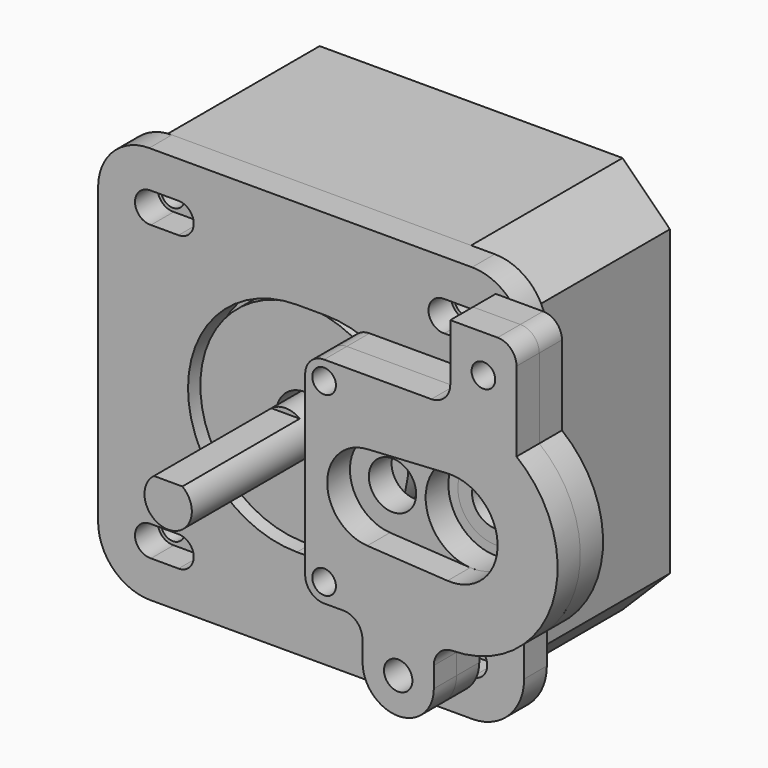
from build123d import *

# Parameters (mm, degrees)
F0_W      = 42
F0_H      = 42
F0_R      = 1.25
F0_R_2    = 11
F0_R_3    = 3
F1_DEPTH  = 20
F2_DEPTH  = 2
F3_SIZE   = 5
F4_R      = 2.5
F5_DEPTH  = 40
F7_DEPTH  = 15.5
F9_DEPTH  = 3
F10_R     = 4
F11_DEPTH = 25
F12_R     = 4
F12_R_2   = 2.5
F13_DEPTH = 2.5
F14_R     = 1.5
F14_R_2   = 2.5
F14_R_3   = 5
F15_DEPTH = 3
F16_R     = 1.5
F17_DEPTH = 3
F18_R     = 1.25
F19_DEPTH = 25


with BuildPart() as f1:
    # F0 (on Front) → F1 (new body)
    with BuildSketch(Plane.XZ):
        Rectangle(F0_W, F0_H)
        with Locations((-15.5, -15.5)):
            Circle(F0_R, mode=Mode.SUBTRACT)
        with Locations((15.5, -15.5)):
            Circle(F0_R, mode=Mode.SUBTRACT)
        with Locations((-15.5, 15.5)):
            Circle(F0_R, mode=Mode.SUBTRACT)
        Circle(F0_R_2, mode=Mode.SUBTRACT)
        with Locations((15.5, 15.5)):
            Circle(F0_R, mode=Mode.SUBTRACT)
        Circle(F0_R_2)
        Circle(F0_R_3, mode=Mode.SUBTRACT)
    extrude(amount=-F1_DEPTH)

    # F0 (on Front) → F2 (join)
    with BuildSketch(Plane.XZ):
        Circle(F0_R_2)
        Circle(F0_R_3, mode=Mode.SUBTRACT)
    extrude(amount=F2_DEPTH)

    # F3
    f3_edges = [f1.edges().sort_by_distance(p)[0] for p in [
        (-21, 10, 21),
        (21, 10, 21),
        (21, 10, -21),
        (-21, 10, -21),
    ]]
    chamfer(f3_edges, length=F3_SIZE)


with BuildPart() as f5:
    # F4 (on face) → F5 (new body)
    with BuildSketch(Plane(origin=(0, 20, 0), x_dir=(-1, 0, 0), z_dir=(0, 1, 0))):
        Circle(F4_R)
    extrude(amount=-F5_DEPTH)

    # F6 (on face) → F7 (cut)
    with BuildSketch(Plane.XZ.offset(20)):
        with BuildLine():
            ThreePointArc((1.5, 2), (0, 2.5), (-1.5, 2))
            Line((-1.5, 2), (1.5, 2))
        make_face()
    extrude(amount=-F7_DEPTH, mode=Mode.SUBTRACT)


with BuildPart() as f9:
    # F8 (on face) → F9 (new body)
    with BuildSketch(Plane.XZ):
        with BuildLine():
            Line((-15.5, -21), (18.5, -21))
            ThreePointArc((18.5, -21), (22.3890872965, -19.3890872965), (24, -15.5))
            Line((24, -15.5), (24, -6.8738635424))
            ThreePointArc((24, -6.8738635424), (28.5, 0), (24, 6.8738635424))
            Line((24, 6.8738635424), (24, 15.5))
            ThreePointArc((24, 15.5), (22.3890872965, 19.3890872965), (18.5, 21))
            Line((18.5, 21), (-15.6, 21))
            ThreePointArc((-15.6, 21), (-19.4183766184, 19.4183766184), (-21, 15.6))
            Line((-21, 15.6), (-21, -15.5))
            ThreePointArc((-21, -15.5), (-19.3890872965, -19.3890872965), (-15.5, -21))
        make_face()
        with BuildLine():
            ThreePointArc((-15.5200249009, -13.9001253164), (-15.500066393, -13.9000000014), (-15.4801078747, -13.90012366))
            Line((-15.4801078747, -13.90012366), (-12.500066393, -13.9000000014))
            ThreePointArc((-12.500066393, -13.9000000014), (-10.9000001196, -15.5006185623), (-12.5013035174, -17.099999469))
            Line((-12.5013035174, -17.099999469), (-15.4128983262, -17.0976273966))
            ThreePointArc((-15.4128983262, -17.0976273966), (-17.0991027833, -15.5535750719), (-15.5200249009, -13.9001253164))
        make_face(mode=Mode.SUBTRACT)
        with BuildLine():
            ThreePointArc((15.4799750991, -13.9001253164), (15.499933607, -13.9000000014), (15.5198921253, -13.90012366))
            Line((15.5198921253, -13.90012366), (18.499933607, -13.9000000014))
            ThreePointArc((18.499933607, -13.9000000014), (20.0999998804, -15.5006185623), (18.4986964826, -17.099999469))
            Line((18.4986964826, -17.099999469), (15.5871016738, -17.0976273966))
            ThreePointArc((15.5871016738, -17.0976273966), (13.9008972167, -15.5535750719), (15.4799750991, -13.9001253164))
        make_face(mode=Mode.SUBTRACT)
        with BuildLine():
            ThreePointArc((3, 11.5), (14.5, 0), (3, -11.5))
            Line((3, -11.5), (0, -11.5))
            ThreePointArc((0, -11.5), (-11.5, 0), (0, 11.5))
            Line((0, 11.5), (3, 11.5))
        make_face(mode=Mode.SUBTRACT)
        with BuildLine():
            ThreePointArc((-15.5200249009, 17.0998746836), (-15.500066393, 17.0999999986), (-15.4801078747, 17.09987634))
            Line((-15.4801078747, 17.09987634), (-12.500066393, 17.0999999986))
            ThreePointArc((-12.500066393, 17.0999999986), (-10.9000001196, 15.4993814377), (-12.5013035174, 13.900000531))
            Line((-12.5013035174, 13.900000531), (-15.4128983262, 13.9023726034))
            ThreePointArc((-15.4128983262, 13.9023726034), (-17.0991027833, 15.4464249281), (-15.5200249009, 17.0998746836))
        make_face(mode=Mode.SUBTRACT)
        with BuildLine():
            ThreePointArc((15.4799750991, 17.0998746836), (15.499933607, 17.0999999986), (15.5198921253, 17.09987634))
            Line((15.5198921253, 17.09987634), (18.499933607, 17.0999999986))
            ThreePointArc((18.499933607, 17.0999999986), (20.0999998804, 15.4993814377), (18.4986964826, 13.900000531))
            Line((18.4986964826, 13.900000531), (15.5871016738, 13.9023726034))
            ThreePointArc((15.5871016738, 13.9023726034), (13.9008972167, 15.4464249281), (15.4799750991, 17.0998746836))
        make_face(mode=Mode.SUBTRACT)
    extrude(amount=F9_DEPTH)

    # F10 (on face) → F11 (cut)
    with BuildSketch(Plane.XZ.offset(3)):
        with Locations((21, 0)):
            Circle(F10_R)
    extrude(amount=-F11_DEPTH, mode=Mode.SUBTRACT)


with BuildPart() as f13:
    # F12 (on face) → F13 (new body)
    with BuildSketch(Plane.XZ.offset(3)):
        with Locations((21, 0)):
            Circle(F12_R)
        with Locations((21, 0)):
            Circle(F12_R_2, mode=Mode.SUBTRACT)
    extrude(amount=-F13_DEPTH)


with BuildPart() as f15:
    # F14 (on face) → F15 (new body)
    with BuildSketch(Plane.XZ.offset(3)):
        with BuildLine():
            Line((5.6725820601, 9.3386074081), (5.6725820601, -9.3386074081))
            ThreePointArc((5.6725820601, -9.3386074081), (6.2583684977, -10.7528209705), (7.6725820601, -11.3386074081))
            Line((7.6725820601, -11.3386074081), (9.7175180337, -11.3386074081))
            ThreePointArc((9.7175180337, -11.3386074081), (11.1253990941, -11.918089573), (11.7174381896, -13.3207364883))
            Line((11.7174381896, -13.3207364883), (11.737212143, -15.5336235823))
            ThreePointArc((11.737212143, -15.5336235823), (15.516811959, -19.2629005249), (19.2629380811, -15.5))
            Line((19.2629380811, -15.5), (19.2629380811, -13.3386074081))
            ThreePointArc((19.2629380811, -13.3386074081), (19.8211268568, -11.9525408897), (21.1841184746, -11.3401611442))
            ThreePointArc((21.1841184746, -11.3401611442), (21.2235206216, -11.3389958799), (21.2629380811, -11.3386074081))
            ThreePointArc((21.2629380811, -11.3386074081), (31.7623537708, -3.5783928938), (28, 8.9237410535))
            Line((28, 8.9237410535), (28, 17.3386074081))
            ThreePointArc((28, 17.3386074081), (27.4142135624, 18.7528209705), (26, 19.3386074081))
            Line((26, 19.3386074081), (21, 19.3386074081))
            Line((21, 19.3386074081), (21, 13.3386074081))
            ThreePointArc((21, 13.3386074081), (20.4142135624, 11.9243938457), (19, 11.3386074081))
            Line((19, 11.3386074081), (7.6725820601, 11.3386074081))
            ThreePointArc((7.6725820601, 11.3386074081), (6.2583684977, 10.7528209705), (5.6725820601, 9.3386074081))
        make_face()
        with Locations((15.5, -15.5)):
            Circle(F14_R, mode=Mode.SUBTRACT)
        with Locations((12.5, 0)):
            Circle(F14_R_2, mode=Mode.SUBTRACT)
        with Locations((21, 0)):
            Circle(F14_R_3, mode=Mode.SUBTRACT)
        with BuildLine():
            ThreePointArc((21.2629380811, -11.3386074081), (21.2235206216, -11.3389958799), (21.1841184746, -11.3401611442))
            ThreePointArc((21.1841184746, -11.3401611442), (21.2235296278, -11.33945276), (21.2629380811, -11.3386074081))
        make_face()
    extrude(amount=F15_DEPTH)


with BuildPart() as f17:
    # F16 (on face) → F17 (new body)
    with BuildSketch(Plane.XZ.offset(6)):
        with BuildLine():
            ThreePointArc((19.2629380811, -13.3386074081), (19.8211268568, -11.9525408897), (21.1841184746, -11.3401611442))
            ThreePointArc((21.1841184746, -11.3401611442), (31.7498522145, -3.6157754018), (28, 8.9237410535))
            Line((28, 8.9237410535), (28, 17.3386074081))
            ThreePointArc((28, 17.3386074081), (27.4142135624, 18.7528209705), (26, 19.3386074081))
            Line((26, 19.3386074081), (21, 19.3386074081))
            Line((21, 19.3386074081), (21, 13.3386074081))
            ThreePointArc((21, 13.3386074081), (20.4142135624, 11.9243938457), (19, 11.3386074081))
            Line((19, 11.3386074081), (7.6725820601, 11.3386074081))
            ThreePointArc((7.6725820601, 11.3386074081), (6.2583684977, 10.7528209705), (5.6725820601, 9.3386074081))
            Line((5.6725820601, 9.3386074081), (5.6725820601, -9.3386074081))
            ThreePointArc((5.6725820601, -9.3386074081), (6.2583684977, -10.7528209705), (7.6725820601, -11.3386074081))
            Line((7.6725820601, -11.3386074081), (9.7175180337, -11.3386074081))
            ThreePointArc((9.7175180337, -11.3386074081), (11.1253990941, -11.918089573), (11.7174381896, -13.3207364883))
            Line((11.7174381896, -13.3207364883), (11.737212143, -15.5336235823))
            ThreePointArc((11.737212143, -15.5336235823), (15.516811959, -19.2629005249), (19.2629380811, -15.5))
            Line((19.2629380811, -15.5), (19.2629380811, -13.3386074081))
        make_face()
        with Locations((15.5, -15.5)):
            Circle(F16_R, mode=Mode.SUBTRACT)
        with BuildLine():
            ThreePointArc((20.7058823529, 4.9913419848), (26, 0), (20.7058823529, -4.9913419848))
            Line((20.7058823529, -4.9913419848), (12.2352941176, -4.4922077864))
            ThreePointArc((12.2352941176, -4.4922077864), (8, 0), (12.2352941176, 4.4922077864))
            Line((12.2352941176, 4.4922077864), (20.7058823529, 4.9913419848))
        make_face(mode=Mode.SUBTRACT)
    extrude(amount=F17_DEPTH)


with BuildPart() as f19_tool:
    # F18 (on face) → F19 (new body)
    with BuildSketch(Plane.XZ.offset(9)):
        with Locations((24.5, 15.3386074081)):
            Circle(F18_R)
        with Locations((7.6725820601, 9.3386074081)):
            Circle(F18_R)
        with Locations((7.6725820601, -9.3386074081)):
            Circle(F18_R)
    extrude(amount=-F19_DEPTH)


with BuildPart() as f15_1:
    add(f15.part)

    # F19: cut by f19_tool
    add(f19_tool.part, mode=Mode.SUBTRACT)


with BuildPart() as f17_1:
    add(f17.part)

    # F19: cut by f19_tool
    add(f19_tool.part, mode=Mode.SUBTRACT)


solid = Compound([f1.part, f5.part, f9.part, f13.part, f15_1.part, f17_1.part])
